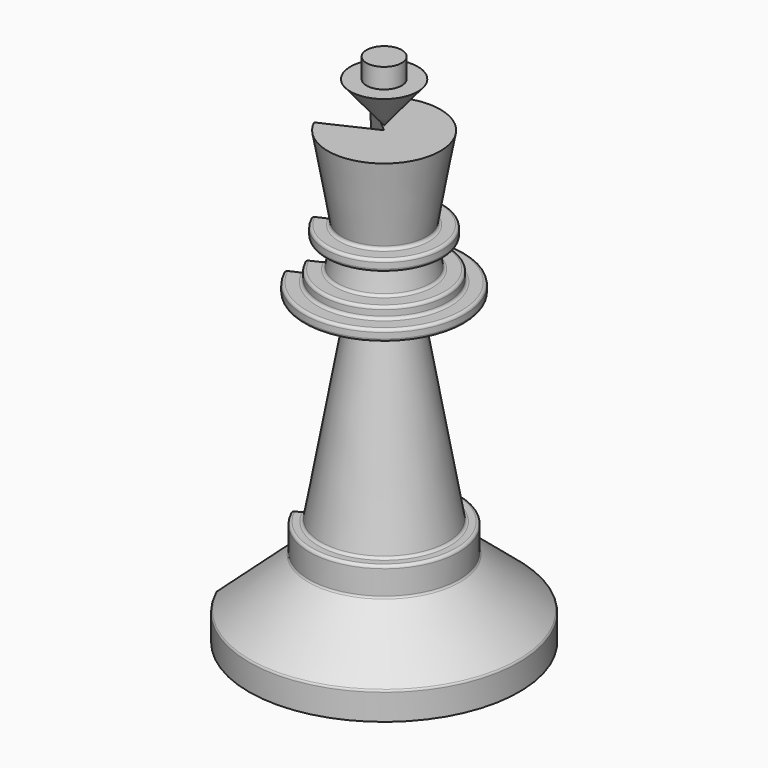
from build123d import *

# Parameters (mm, degrees)
F1_ANGLE_START = 25
F1_ANGLE       = 295
F2_W           = 1.9843422342
F2_H           = 2.2462382913


# Not quite as in the source:
# - a feature of the source that left no trace in its solid (it failed there, or was rolled back) is left out


with BuildPart() as f1:
    # F0 (on Front) → F1 (revolve)
    with BuildSketch(Plane.XZ, mode=Mode.PRIVATE) as f1_sk:
        with BuildLine():
            Line((-15.24, 0), (0, 0))
            Line((0, 0), (0, 50.8))
            Line((0, 50.8), (-6.35, 50.8))
            Line((-6.35, 50.8), (-4.7617064118, 41.792339449))
            ThreePointArc((-4.7617064118, 41.792339449), (-4.8311637627, 41.5331210865), (-5.0743828734, 41.4197061526))
            Line((-5.0743828734, 41.4197061526), (-6.2835011077, 41.4197061526))
            ThreePointArc((-6.2835011077, 41.4197061526), (-6.5080075107, 41.3267125556), (-6.6010011077, 41.1022061526))
            Line((-6.6010011077, 41.1022061526), (-6.6010011077, 40.4672061526))
            ThreePointArc((-6.6010011077, 40.4672061526), (-6.5080075107, 40.2426997495), (-6.2835011077, 40.1497061526))
            Line((-6.2835011077, 40.1497061526), (-5.0743828734, 40.1497061526))
            ThreePointArc((-5.0743828734, 40.1497061526), (-4.8311637627, 40.0362912186), (-4.7617064118, 39.7770728561))
            Line((-4.7617064118, 39.7770728561), (-5.2010717431, 37.2853082403))
            ThreePointArc((-5.2010717431, 37.2853082403), (-5.3096631386, 37.0972224261), (-5.5137482047, 37.0229415367))
            Line((-5.5137482047, 37.0229415367), (-6.8348340718, 37.0229415367))
            ThreePointArc((-6.8348340718, 37.0229415367), (-7.0593404748, 36.9299479398), (-7.1523340718, 36.7054415367))
            Line((-7.1523340718, 36.7054415367), (-7.1523340718, 36.0704415367))
            ThreePointArc((-7.1523340718, 36.0704415367), (-7.2453276688, 35.8459351337), (-7.4698340718, 35.7529415367))
            Line((-7.4698340718, 35.7529415367), (-8.7398340718, 35.7529415367))
            ThreePointArc((-8.7398340718, 35.7529415367), (-8.9643404748, 35.6599479398), (-9.0573340718, 35.4354415367))
            Line((-9.0573340718, 35.4354415367), (-9.0573340718, 34.8004415367))
            ThreePointArc((-9.0573340718, 34.8004415367), (-8.9643404748, 34.5759351337), (-8.7398340718, 34.4829415367))
            Line((-8.7398340718, 34.4829415367), (-3.5686493249, 34.4829415367))
            ThreePointArc((-3.5686493249, 34.4829415367), (-3.3254302142, 34.3695266028), (-3.2559728633, 34.1103082403))
            Line((-3.2559728633, 34.1103082403), (-7.113602572, 12.2326030065))
            ThreePointArc((-7.113602572, 12.2326030065), (-7.2221939675, 12.0445171922), (-7.4262790336, 11.9702363029))
            Line((-7.4262790336, 11.9702363029), (-8.1123649007, 11.9702363029))
            ThreePointArc((-8.1123649007, 11.9702363029), (-8.3368713037, 11.8772427059), (-8.4298649007, 11.6527363029))
            Line((-8.4298649007, 11.6527363029), (-8.4298649007, 8.9432889844))
            ThreePointArc((-8.4298649007, 8.9432889844), (-8.4596121783, 8.8091076862), (-8.5432798346, 8.7000698737))
            Line((-8.5432798346, 8.7000698737), (-15.1265850661, 3.176020882))
            ThreePointArc((-15.1265850661, 3.176020882), (-15.2102527224, 3.0669830694), (-15.24, 2.9328017713))
            Line((-15.24, 2.9328017713), (-15.24, 0))
        make_face()
    revolve(f1_sk.sketch.rotate(Axis((0, 0, 25.4), (0, 0, 1)), F1_ANGLE_START), axis=Axis((0, 0, 25.4), (0, 0, 1)), revolution_arc=F1_ANGLE)


with BuildPart() as f3:
    # F2 (on Right) → F3 (revolve)
    with BuildSketch(Plane.YZ):
        Polygon((-3.8027237169, 55.8756142855), (0, 51.2761808932), (0, 55.8756142855), (-1.9843422342, 55.8756142855), align=None)
        with Locations((-0.9921711171, 56.9987334311)):
            Rectangle(F2_W, F2_H)
    revolve(axis=Axis((0, 0, 56.9987334311), (0, 0, 1)))


solid = Compound([f1.part, f3.part])
